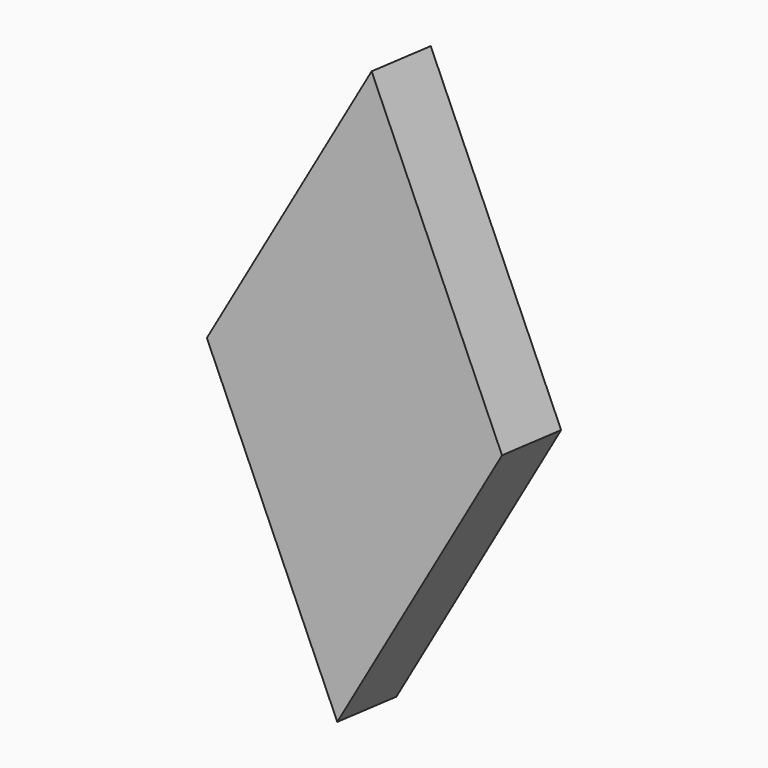
from build123d import *

# Parameters (mm, degrees)
F1_DEPTH = 2
F6_DEPTH = 2


with BuildPart() as f1:
    # F0 (on Front) → F1 (new body)
    with BuildSketch(Plane.XZ):
        Polygon((5.1576569676, 2.7410463956), (0, 0), (5.1576569676, -2.7410463956), (10.3153139353, 0), align=None)
    extrude(amount=F1_DEPTH)


with BuildPart() as f6:
    # F5 (on face) → F6 (new body)
    with BuildSketch(Plane(origin=(-2.1093194974, -51.3742344161, 3.9689756511), x_dir=(-0.9991631758, 0.0407801704, -0.003150519), z_dir=(0.0409016879, 0.9961946981, -0.0769621688))):
        Polygon((0, 7.8918055439), (-4.3265928001, 0), (0, -7.8918055439), (4.3265928001, 0), align=None)
    extrude(amount=-F6_DEPTH)


solid = f6.part
